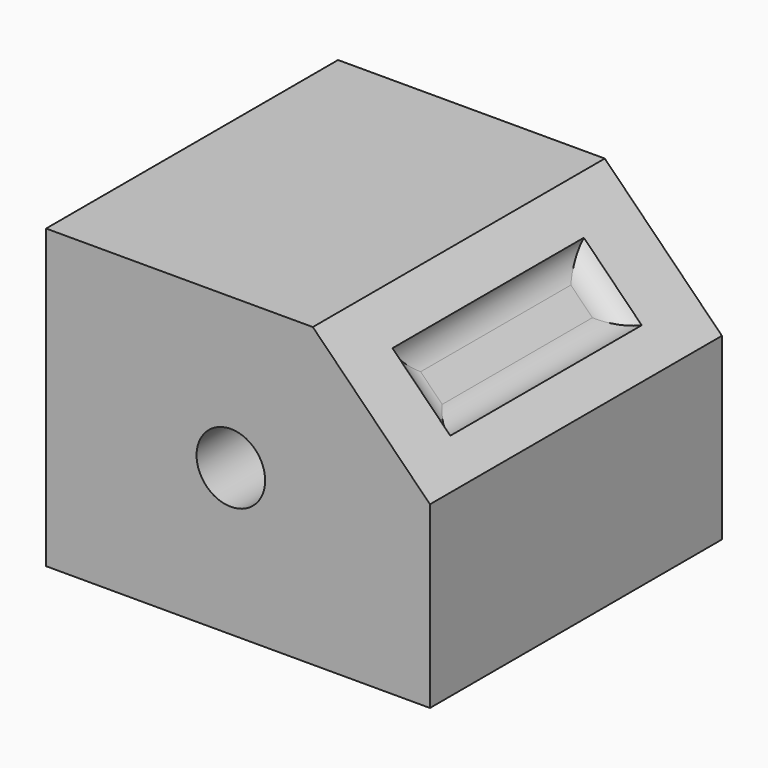
from build123d import *

# Parameters (mm, degrees)
F0_W        = 65.5969455838
F0_H        = 62.3628050089
F1_DEPTH    = 50.8
F3_DEPTH    = 101.6
F4_W        = 40.8792179078
F4_H        = 14.0294057783
F5_DEPTH    = 2.54
F6_R        = 5.8595306003
F7_DEPTH    = 25.4
F8_T1_DEPTH = 51.8777405358
F8_T3_DEPTH = 14.0294057783
F8_T5_DEPTH = 14.0294057783


# Not quite as in the source:
# - a fillet or chamfer that OpenCascade refuses, or shapes differently, is made with other operations: its cross-section is extruded or revolved along the edge and cut away or added


with BuildPart() as f1:
    # F0 (on Top) → F1 (new body)
    with BuildSketch(Plane.XY):
        with Locations((32.7984727919, 31.1814025044)):
            Rectangle(F0_W, F0_H)
    extrude(amount=F1_DEPTH)

    # F2 (on face) → F3 (cut)
    with BuildSketch(Plane.XZ):
        Polygon((89.7827520967, 45.4889908433), (33.5367023945, 62.9252642393), (74.5963230729, 21.5844195336), align=None)
    extrude(amount=-F3_DEPTH, mode=Mode.SUBTRACT)

    # F4 (on face) → F5 (cut)
    with BuildSketch(Plane(origin=(48.3447062482, 0, 48.0158379562), x_dir=(0, 1, 0), z_dir=(0.7095159293, 0, 0.7046893969))):
        with Locations((30.5939735845, -10.8757299604)):
            Rectangle(F4_W, F4_H)
    extrude(amount=-F5_DEPTH, mode=Mode.SUBTRACT)

    # F6 (on face) → F7 (cut)
    with BuildSketch(Plane.XZ):
        with Locations((31.5736755729, 25.0635799021)):
            Circle(F6_R)
    extrude(amount=-F7_DEPTH, mode=Mode.SUBTRACT)

    # F8: fillet of radius 5.08 on 4 edges, made by hand

    # F8_s2 → F8_t1 (join)
    with BuildSketch(Plane.XZ.offset(-62.0321051664)):
        with BuildLine():
            ThreePointArc((51.0655310864, 45.2763777457), (51.0565565883, 42.6467915619), (52.3635775369, 40.3650158763))
            Line((52.3635775369, 40.3650158763), (49.263360626, 43.4864666776))
            Line((49.263360626, 43.4864666776), (51.0655310864, 45.2763777457))
        make_face()
        with BuildLine():
            ThreePointArc((60.9519045829, 35.3222908675), (58.3223183991, 35.3312653655), (56.0495172115, 36.6538306007))
            Line((56.0495172115, 36.6538306007), (59.1497341225, 33.5323797994))
            Line((59.1497341225, 33.5323797994), (60.9519045829, 35.3222908675))
        make_face()
    extrude(amount=F8_T1_DEPTH)

    # F8_s4 → F8_t3 (join)
    with BuildSketch(Plane(origin=(12.6071983347, 0, -12.6935470887), x_dir=(0, 1, 0), z_dir=(-0.7046893969, 0, 0.7095159293))):
        with BuildLine():
            ThreePointArc((51.0335825384, -68.1375910703), (49.1741734871, -66.278182019), (46.6341734871, -65.5975910703))
            Line((46.6341734871, -65.5975910703), (51.0335825384, -65.5975910703))
            Line((51.0335825384, -65.5975910703), (51.0335825384, -68.1375910703))
        make_face()
    extrude(amount=F8_T3_DEPTH)

    # F8_s6 → F8_t5 (join)
    with BuildSketch(Plane(origin=(2.7208248382, 0, -2.7394602105), x_dir=(0, 1, 0), z_dir=(0.7046893969, 0, -0.7095159293))):
        with BuildLine():
            ThreePointArc((10.1543646306, 68.1375910703), (12.0137736818, 66.278182019), (14.5537736818, 65.5975910703))
            Line((14.5537736818, 65.5975910703), (10.1543646306, 65.5975910703))
            Line((10.1543646306, 65.5975910703), (10.1543646306, 68.1375910703))
        make_face()
    extrude(amount=F8_T5_DEPTH)


solid = f1.part
